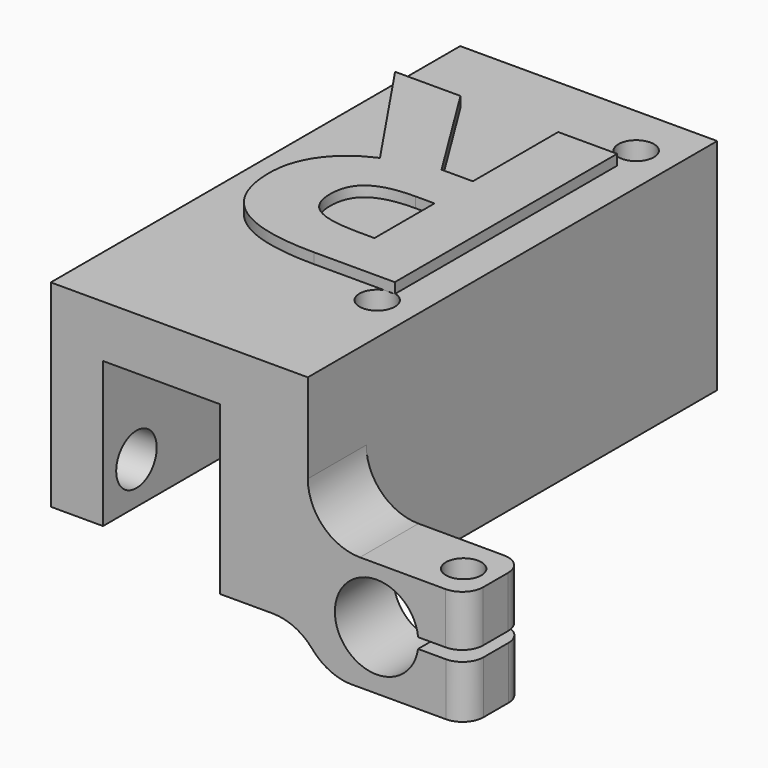
from build123d import *

# Parameters (mm, degrees)
F1_DEPTH      = 7
F2_DEPTH      = 42
F3_R          = 1.7
F3_R_2        = 11
F4_DEPTH      = 21.001
F5_R          = 4
F6_DEPTH      = 10
F7_DEPTH      = 21.001
F8_R          = 1.4
F9_DEPTH      = 11.0191891876
F8_R_2        = 1.7
F10_DEPTH     = 4.9110969969
F11_R         = 5
F12_R         = 5
F13_R         = 5
F14_R         = 2
F15_R         = 2.2
F15_R_2       = 2.4255023423
F16_DEPTH     = 6
F17_TEXT_SIZE = 37.2792890351
F18_DEPTH     = 1


# Not quite as in the source:
# - a feature names something its author has since deleted; it is built from what else it names
# - Text() gives the source's letters only with a copy of the font that has no kerning and outlines rounded to 1/6400 em; it was checked with that copy


with BuildPart() as f1:
    # F0 (on Front) → F1 (new body)
    with BuildSketch(Plane.XZ):
        Polygon((-18.6721007523, 29.8099789735), (-18.6721007523, 10.8925135386), (-13.6721007523, 10.8925135386), (-13.6721007523, 24.8099789735), (-2.4721007523, 24.8099789735), (-2.4721007523, 8.8099789735), (5.9380548998, 8.8099789735), (5.9380548998, 16.2656020473), (5.9380548998, 29.8099789735), align=None)
        Polygon((21.1263195603, 16.2417280634), (5.9380548998, 16.2656020473), (5.9380548998, 8.8099789735), (7.3533044869, 5.2860832236), (21.1553367778, 5.2860832236), (21.1553367778, 10.343908232), (14.4860510706, 10.343908232), (14.4860510706, 11.3388913612), (21.1263195603, 11.3388913612), align=None)
    extrude(amount=F1_DEPTH)

    # F0 (on Front) → F2 (join)
    with BuildSketch(Plane.XZ):
        Polygon((-18.6721007523, 29.8099789735), (-18.6721007523, 10.8925135386), (-13.6721007523, 10.8925135386), (-13.6721007523, 24.8099789735), (-2.4721007523, 24.8099789735), (-2.4721007523, 8.8099789735), (5.9380548998, 8.8099789735), (5.9380548998, 16.2656020473), (5.9380548998, 29.8099789735), align=None)
    extrude(amount=-F2_DEPTH)

    # F3 (on face) → F4 (cut, through all)
    with BuildSketch(Plane(origin=(0, 0, 8.8099789735), x_dir=(1, 0, 0), z_dir=(0, 0, -1))):
        with Locations((2.1850741468, -6)):
            Circle(F3_R)
        with Locations((2.1850741468, -37)):
            Circle(F3_R)
        with Locations((17.6850741468, -21.5)):
            Circle(F3_R_2)
    extrude(amount=-F4_DEPTH, mode=Mode.SUBTRACT)

    # F5 (on face) → F6 (cut)
    with BuildSketch(Plane.XZ.offset(7)):
        with Locations((12.5278992477, 10.8989789735)):
            Circle(F5_R)
    extrude(amount=-F6_DEPTH, mode=Mode.SUBTRACT)

    # F3 (on face) → F7 (cut, through all)
    with BuildSketch(Plane(origin=(0, 0, 8.8099789735), x_dir=(1, 0, 0), z_dir=(0, 0, -1))):
        with Locations((2.1850741468, -6)):
            Circle(F3_R)
        with Locations((2.1850741468, -37)):
            Circle(F3_R)
        with Locations((17.6850741468, -21.5)):
            Circle(F3_R_2)
    extrude(amount=-F7_DEPTH, mode=Mode.SUBTRACT)

    # F8 (on face) → F9 (cut, through all)
    with BuildSketch(Plane(origin=(0.0255820271, 0, 16.2748956885), x_dir=(0.9999987646, 0, -0.0015718685), z_dir=(0.0015718685, 0, 0.9999987646))):
        with Locations((18.1007636008, -3.5767070949)):
            Circle(F8_R)
    extrude(amount=-F9_DEPTH, mode=Mode.SUBTRACT)

    # F8 (on face) → F10 (cut, through all)
    with BuildSketch(Plane(origin=(0.0255820271, 0, 16.2748956885), x_dir=(0.9999987646, 0, -0.0015718685), z_dir=(0.0015718685, 0, 0.9999987646))):
        with Locations((18.1007636008, -3.5767070949)):
            Circle(F8_R_2)
        with Locations((18.1007636008, -3.5767070949)):
            Circle(F8_R, mode=Mode.SUBTRACT)
    extrude(amount=-F10_DEPTH, mode=Mode.SUBTRACT)

    # F11
    f11_edges = [f1.edges().sort_by_distance(p)[0] for p in [
        (5.938055, -3.5, 16.265602),
    ]]
    fillet(f11_edges, radius=F11_R)

    # F12
    f12_edges = [f1.edges().sort_by_distance(p)[0] for p in [
        (5.938055, -3.5, 8.809979),
    ]]
    fillet(f12_edges, radius=F12_R)

    # F13
    f13_edges = [f1.edges().sort_by_distance(p)[0] for p in [
        (7.353304, -3.5, 5.286083),
    ]]
    fillet(f13_edges, radius=F13_R)

    # F14
    f14_edges = [f1.edges().sort_by_distance(p)[0] for p in [
        (21.12632, -7, 13.79031),
        (21.155337, -7, 7.814996),
        (21.12632, 0, 13.79031),
        (21.155337, 0, 7.814996),
    ]]
    fillet(f14_edges, radius=F14_R)

    # F15 (on face) → F16 (cut)
    with BuildSketch(Plane(origin=(-18.6721007523, 0, 0), x_dir=(0, -1, 0), z_dir=(-1, 0, 0))):
        with Locations((-38, 14.8925135386)):
            Circle(F15_R)
        with Locations((3, 14.8925135386)):
            Circle(F15_R_2)
    extrude(amount=-F16_DEPTH, mode=Mode.SUBTRACT)

    # F17 (on face) → F18 (join)
    with BuildSketch(Plane.XY.offset(29.8099789735)):
        with Locations(Location((5.9380548998, 34.2090676236), (0, 0, 180))):
            Text('R', F17_TEXT_SIZE, font='Open Sans', font_style=FontStyle.BOLD, text_align=(TextAlign.LEFT, TextAlign.BOTTOM))
    extrude(amount=F18_DEPTH)


solid = f1.part
